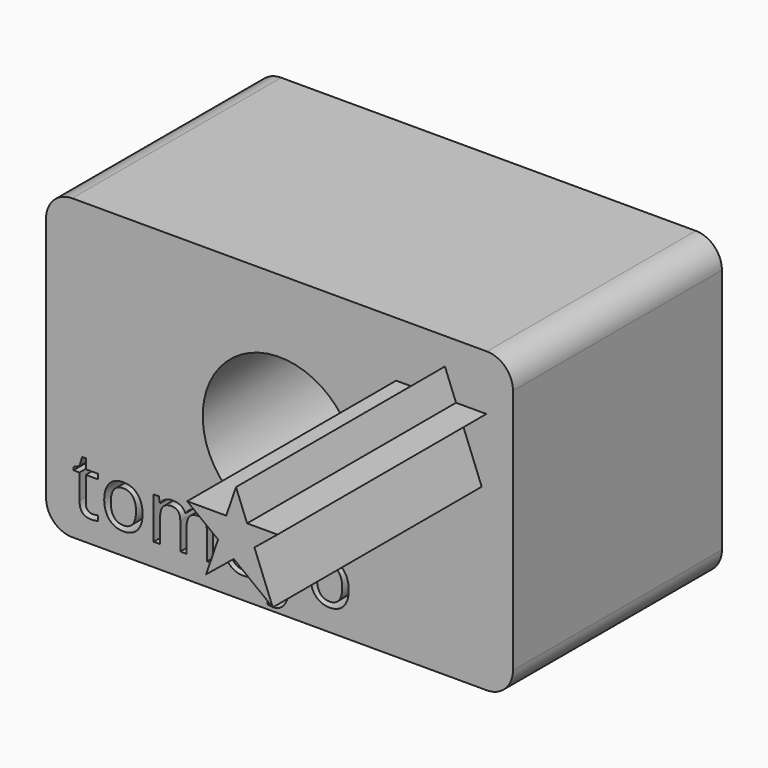
from build123d import *

# Parameters (mm, degrees)
F0_W          = 90.8156037331
F0_H          = 58.034569025
F1_DEPTH      = 50.8
F3_R          = 14.9414754822
F4_DEPTH      = 127
F5_R          = 5.08
F6_R          = 5.08
F7_R          = 5.08
F8_R          = 5.08
F10_DEPTH     = 50.8
F11_TEXT_SIZE = 15.1764045263
F12_DEPTH     = 25.4


# Not quite as in the source:
# - Text() gives the source's letters only with a copy of the font that has no kerning and outlines rounded to 1/6400 em; it was checked with that copy


with BuildPart() as f1:
    # F0 (on Front) → F1 (new body)
    with BuildSketch(Plane.XZ):
        Rectangle(F0_W, F0_H)
    extrude(amount=F1_DEPTH)

    # F3 (on face) → F4 (cut)
    with BuildSketch(Plane.XZ.offset(50.8)):
        Circle(F3_R)
    extrude(amount=-F4_DEPTH, mode=Mode.SUBTRACT)

    # F5
    f5_edges = [f1.edges().sort_by_distance(p)[0] for p in [
        (45.407802, -25.4, 29.017285),
    ]]
    fillet(f5_edges, radius=F5_R)

    # F6
    f6_edges = [f1.edges().sort_by_distance(p)[0] for p in [
        (45.407802, -25.4, -29.017285),
    ]]
    fillet(f6_edges, radius=F6_R)

    # F7
    f7_edges = [f1.edges().sort_by_distance(p)[0] for p in [
        (-45.407802, -25.4, 29.017285),
    ]]
    fillet(f7_edges, radius=F7_R)

    # F8
    f8_edges = [f1.edges().sort_by_distance(p)[0] for p in [
        (-45.407802, -25.4, -29.017285),
    ]]
    fillet(f8_edges, radius=F8_R)

    # F9 (on face) → F10 (join)
    with BuildSketch(Plane.XZ.offset(50.8)):
        Polygon((30.2691630844, 18.2783100754), (22.6789172739, 18.2783100754), (28.6794948687, 13.6766399491), align=None)
        Polygon((32.1736857295, 23.7914007157), (30.2691630844, 18.2783100754), (34.329642351, 18.2783100754), align=None)
        Polygon((34.329642351, 18.2783100754), (30.2691630844, 18.2783100754), (28.6794948687, 13.6766399491), (31.7324881306, 11.3353873502), (35.7594464529, 14.622095691), align=None)
        Polygon((31.7324881306, 11.3353873502), (28.6794948687, 13.6766399491), (26.3543110341, 6.9458461367), align=None)
        Polygon((40.2391329408, 18.2783100754), (34.329642351, 18.2783100754), (35.7594464529, 14.622095691), align=None)
        Polygon((35.7594464529, 14.622095691), (31.7324881306, 11.3353873502), (39.3202826381, 5.5165262893), align=None)
    extrude(amount=F10_DEPTH)

    # F11 (on face) → F12 (cut)
    with BuildSketch(Plane.XZ.offset(50.8)):
        with Locations((-40.3085276484, -24.6464796364)):
            Text('tomoyo', F11_TEXT_SIZE, font='Open Sans', text_align=(TextAlign.LEFT, TextAlign.BOTTOM))
    extrude(amount=-F12_DEPTH, mode=Mode.SUBTRACT)


solid = f1.part
